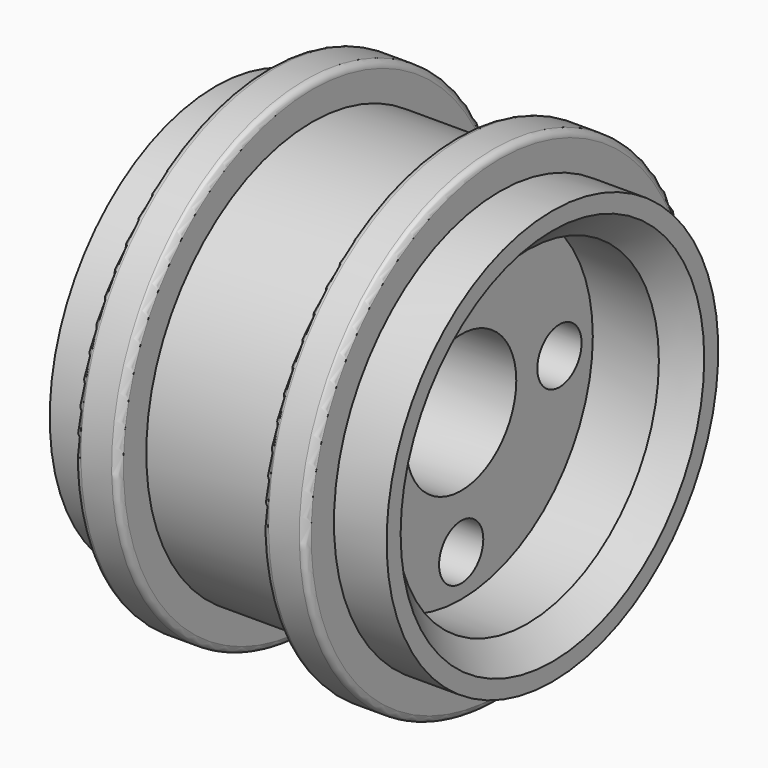
from build123d import *

# Parameters (mm, degrees)
F2_R          = 0.1905
F3_SIZE       = 0.762
F4_R          = 0.8001
F4_R_2        = 1.9939
F5_DEPTH      = 7.3634
F6_R          = 4.7625
F7_DEPTH      = 0.254
F7_DEPTH_BACK = 2.3886


with BuildPart() as f1:
    # F0 (on Front) → F1 (revolve)
    with BuildSketch(Plane.XZ):
        with BuildLine():
            Line((-1.0126, 2.25), (-1.0126, 1))
            Line((-1.0126, 1), (2.4874, 1))
            Line((2.4874, 1), (2.4874, 4.23))
            Line((2.4874, 4.23), (2.9874, 4.73))
            Line((2.9874, 4.73), (4.875, 4.73))
            Line((4.875, 4.73), (4.875, 6))
            Line((4.875, 6), (3.351, 6))
            Line((3.351, 6), (3.351, 7.016))
            Line((3.351, 7.016), (2.081, 7.016))
            Line((2.081, 7.016), (2.081, 6))
            Line((2.081, 6), (-2.081, 6))
            Line((-2.081, 6), (-2.081, 7.016))
            Line((-2.081, 7.016), (-3.351, 7.016))
            Line((-3.351, 7.016), (-3.351, 6))
            Line((-3.351, 6), (-4.875, 6))
            Line((-4.875, 6), (-4.875, 4.73))
            Line((-4.875, 4.73), (-0.0126, 4.73))
            ThreePointArc((-0.0126, 4.73), (0.3409533906, 4.5835533906), (0.4874, 4.23))
            Line((0.4874, 4.23), (0.4874, 3.1160254038))
            Line((0.4874, 3.1160254038), (-1.0126, 2.25))
        make_face()
    revolve(axis=Axis((17.3129402101, 0, 0), (1, 0, 0)))

    # F2
    f2_edges = [f1.edges().sort_by_distance(p)[0] for p in [
        (3.351, 0, -7.016),
        (-2.081, 0, -7.016),
        (2.081, 0, -7.016),
        (-3.351, 0, -7.016),
        (-3.351, 0, -6),
    ]]
    fillet(f2_edges, radius=F2_R)

    # F3
    f3_edges = [f1.edges().sort_by_distance(p)[0] for p in [
        (4.875, 0, -4.73),
        (-4.875, 0, -4.73),
    ]]
    chamfer(f3_edges, length=F3_SIZE)

    # F4 (on face) → F5 (cut, through all)
    with BuildSketch(Plane.YZ.offset(2.4874)):
        with Locations((0, 3.556)):
            Circle(F4_R)
        with Locations((0, -3.556)):
            Circle(F4_R)
        with Locations((-3.556, 0)):
            Circle(F4_R)
        with Locations((3.556, 0)):
            Circle(F4_R)
        Circle(F4_R_2)
    extrude(amount=-F5_DEPTH, mode=Mode.SUBTRACT)

    # F6 (on face) → F7 (cut, two sides)
    with BuildSketch(Plane.YZ.offset(2.4874)) as f7_sk:
        Circle(F6_R)
    extrude(amount=-F7_DEPTH, mode=Mode.SUBTRACT)
    extrude(f7_sk.sketch, amount=F7_DEPTH_BACK, mode=Mode.SUBTRACT)


solid = f1.part
